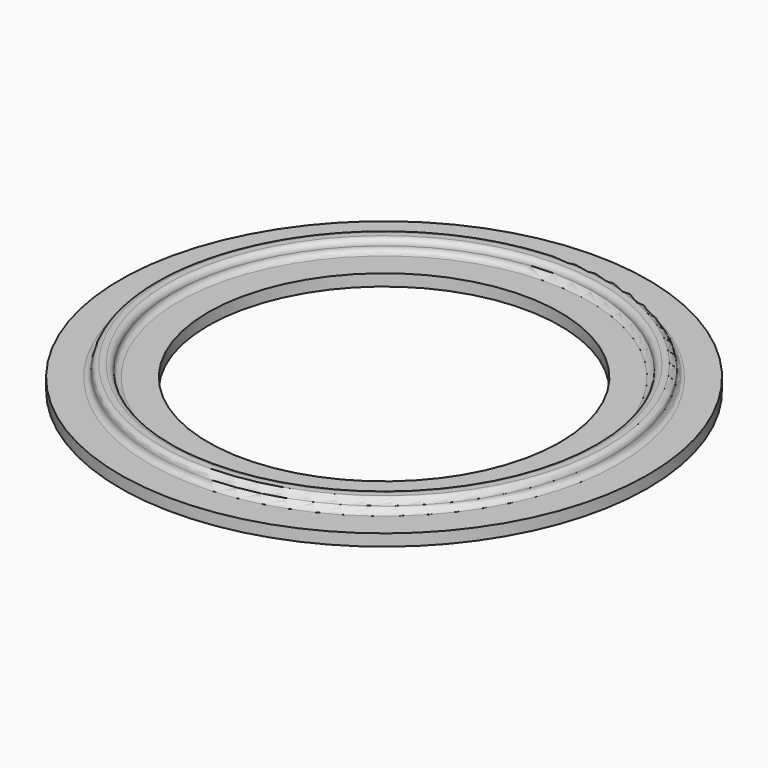
from build123d import *

# Parameters (mm, degrees)
F0_R     = 45
F0_R_2   = 30
F1_DEPTH = 2
F2_R     = 39
F2_R_2   = 36
F3_DEPTH = 2
F4_R     = 0.99999


# Not quite as in the source:
# - a fillet or chamfer is up to 0.001 mm smaller than in the source, because OpenCascade refuses the exact size


with BuildPart() as f1:
    # F0 (on Top) → F1 (new body)
    with BuildSketch(Plane.XY):
        Circle(F0_R)
        Circle(F0_R_2, mode=Mode.SUBTRACT)
    extrude(amount=F1_DEPTH)

    # F2 (on face) → F3 (join)
    with BuildSketch(Plane.XY.offset(2)):
        Circle(F2_R)
        Circle(F2_R_2, mode=Mode.SUBTRACT)
    extrude(amount=F3_DEPTH)

    # F4 (radius 1 in the source; OpenCascade refuses exactly that, so slightly less here)
    f4_edges = [f1.edges().sort_by_distance(p)[0] for p in [
        (-39, 0, 2),
        (-39, 0, 4),
        (-36, 0, 4),
        (-36, 0, 2),
    ]]
    fillet(f4_edges, radius=F4_R)


solid = f1.part
